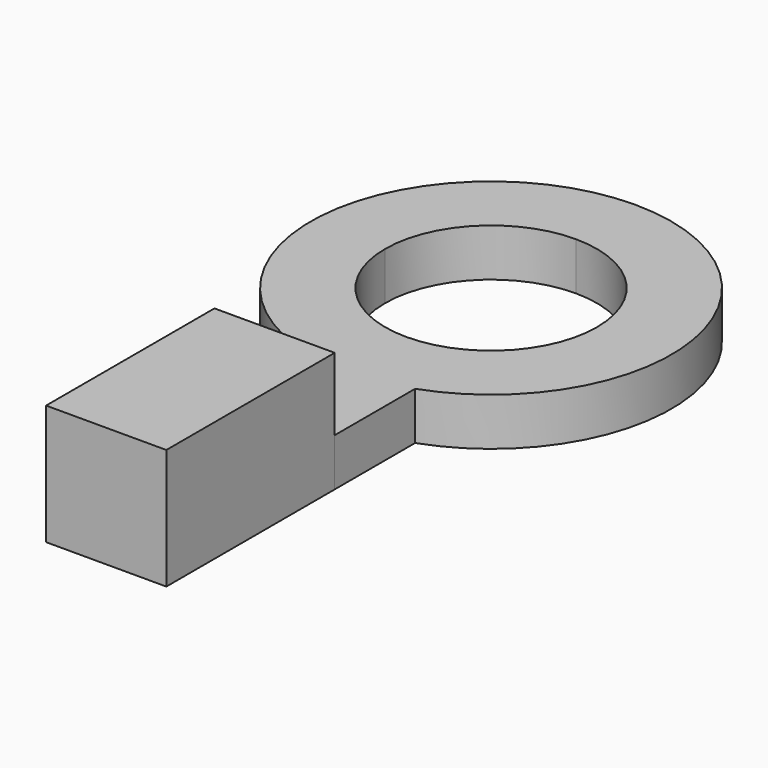
from build123d import *

# Parameters (mm, degrees)
F1_DEPTH = 1.5875
F2_W     = 2
F2_H     = 7
F3_DEPTH = 4


# Not quite as in the source:
# - ends of sketch curves that miss each other by under 0.0002 mm in the source are joined


with BuildPart() as f1:
    # F0 (on Top) → F1 (new body)
    with BuildSketch(Plane.XY):
        with BuildLine():
            Line((-3.52345, 0), (-6, 0))
            ThreePointArc((-6, 0), (-4.8989795096, -3.4641015812), (-2.0000000784, -5.6568542218))
            Line((-2.0000000784, -5.6568542218), (-2, -9))
            Line((-2, -9), (0, -9))
            Line((0, -9), (0, -3.52345))
            ThreePointArc((0, -3.52345), (-2.4914553882, -2.4914553882), (-3.52345, 0))
        make_face()
        with BuildLine():
            ThreePointArc((2.0000000784, -5.6568542218), (4.8989795096, -3.4641015812), (6, 0))
            Line((6, 0), (3.52345, 0))
            ThreePointArc((3.52345, 0), (2.4914553882, -2.4914553882), (0, -3.52345))
            Line((0, -3.52345), (0, -9))
            Line((0, -9), (2, -9))
            Line((2, -9), (2.0000000784, -5.6568542218))
        make_face()
        with BuildLine():
            ThreePointArc((6, 0), (4.2426406871, 4.2426406871), (0, 6))
            Line((0, 6), (0, 3.52345))
            ThreePointArc((0, 3.52345), (2.4914553882, 2.4914553882), (3.52345, 0))
            Line((3.52345, 0), (6, 0))
        make_face()
        with BuildLine():
            Line((0, 3.52345), (0, 6))
            ThreePointArc((0, 6), (-4.2426406871, 4.2426406871), (-6, 0))
            Line((-6, 0), (-3.52345, 0))
            ThreePointArc((-3.52345, 0), (-2.4914553882, 2.4914553882), (0, 3.52345))
        make_face()
    extrude(amount=F1_DEPTH)

    # F2 (on Top) → F3 (join)
    with BuildSketch(Plane.XY):
        with Locations((-1, -12.5)):
            Rectangle(F2_W, F2_H)
        with Locations((1, -12.5)):
            Rectangle(F2_W, F2_H)
    extrude(amount=F3_DEPTH)


solid = f1.part
